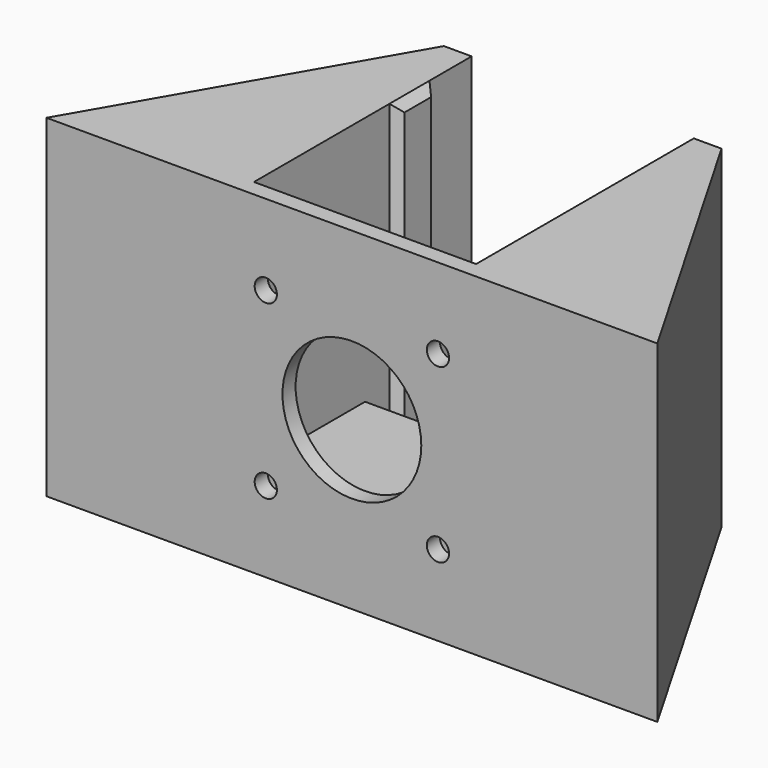
from build123d import *

# Parameters (mm, degrees)
F1_DEPTH  = 60
F2_W      = 40
F2_H      = 20
F3_DEPTH  = 55
F4_W      = 40
F4_H      = 45
F5_DEPTH  = 4
F6_W      = 40
F6_H      = 45
F7_DEPTH  = 25
F8_R      = 12.5
F8_R_2    = 2
F9_DEPTH  = 2.9615242271
F10_W     = 9
F10_H     = 1.5
F10_W_2   = 1.5
F10_H_2   = 9
F11_DEPTH = 10
F12_DEPTH = 45
F13_SIZE  = 1.49999


# Not quite as in the source:
# - a fillet or chamfer is up to 0.001 mm smaller than in the source, because OpenCascade refuses the exact size


with BuildPart() as f1:
    # F0 (on Top) → F1 (new body)
    with BuildSketch(Plane.XY):
        Polygon((30, 51.9615242271), (0, 0), (110, 0), (80, 51.9615242271), align=None)
    extrude(amount=F1_DEPTH)

    # F2 (on face) → F3 (cut)
    with BuildSketch(Plane.XY.offset(60)):
        with Locations((55, 37.9615242271)):
            Rectangle(F2_W, F2_H)
    extrude(amount=-F3_DEPTH, mode=Mode.SUBTRACT)

    # F4 (on face) → F5 (cut, through all)
    with BuildSketch(Plane(origin=(0, 51.9615242271, 0), x_dir=(-1, 0, 0), z_dir=(0, 1, 0))):
        with Locations((-55, 37.5)):
            Rectangle(F4_W, F4_H)
    extrude(amount=-F5_DEPTH, mode=Mode.SUBTRACT)

    # F6 (on face) → F7 (cut)
    with BuildSketch(Plane(origin=(0, 27.9615242271, 0), x_dir=(-1, 0, 0), z_dir=(0, 1, 0))):
        with Locations((-55, 37.5)):
            Rectangle(F6_W, F6_H)
    extrude(amount=-F7_DEPTH, mode=Mode.SUBTRACT)

    # F8 (on face) → F9 (cut, through all)
    with BuildSketch(Plane.XZ):
        with Locations((55, 30)):
            Circle(F8_R)
        with Locations((70.5, 45.5)):
            Circle(F8_R_2)
        with Locations((39.5, 45.5)):
            Circle(F8_R_2)
        with Locations((39.5, 14.5)):
            Circle(F8_R_2)
        with Locations((70.5, 14.5)):
            Circle(F8_R_2)
    extrude(amount=-F9_DEPTH, mode=Mode.SUBTRACT)

    # F10 (on face) → F11 (join, through all)
    with BuildSketch(Plane.XY.offset(15)):
        with Locations((45, 47.2115242271)):
            Rectangle(F10_W, F10_H)
        with Locations((65, 47.2115242271)):
            Rectangle(F10_W, F10_H)
        with Locations((45, 28.7115242271)):
            Rectangle(F10_W, F10_H)
        with Locations((65, 28.7115242271)):
            Rectangle(F10_W, F10_H)
        with Locations((35.75, 37.9615242271)):
            Rectangle(F10_W_2, F10_H_2)
        with Locations((74.25, 37.9615242271)):
            Rectangle(F10_W_2, F10_H_2)
    extrude(amount=-F11_DEPTH)

    # F12 (add, through all): faces of the model
    f12_faces = [f1.faces().sort_by_distance(p)[0] for p in [
        (74.25, 37.9615242271, 15),
        (35.75, 37.9615242271, 15),
    ]]
    extrude(f12_faces, amount=F12_DEPTH)

    # F13 (size 1.5 in the source; OpenCascade refuses exactly that, so slightly less here)
    f13_edges = [f1.edges().sort_by_distance(p)[0] for p in [
        (36.5, 33.461524, 32.5),
        (73.5, 37.961524, 60),
        (73.5, 42.461524, 32.5),
        (36.5, 37.961524, 60),
        (36.5, 42.461524, 32.5),
        (73.5, 33.461524, 32.5),
        (65, 29.461524, 15),
        (69.5, 29.461524, 10),
        (60.5, 29.461524, 10),
        (49.5, 29.461524, 10),
        (45, 29.461524, 15),
        (40.5, 46.461524, 10),
        (45, 46.461524, 15),
        (60.5, 46.461524, 10),
        (65, 46.461524, 15),
        (49.5, 46.461524, 10),
        (40.5, 29.461524, 10),
        (69.5, 46.461524, 10),
    ]]
    chamfer(f13_edges, length=F13_SIZE)


solid = f1.part
